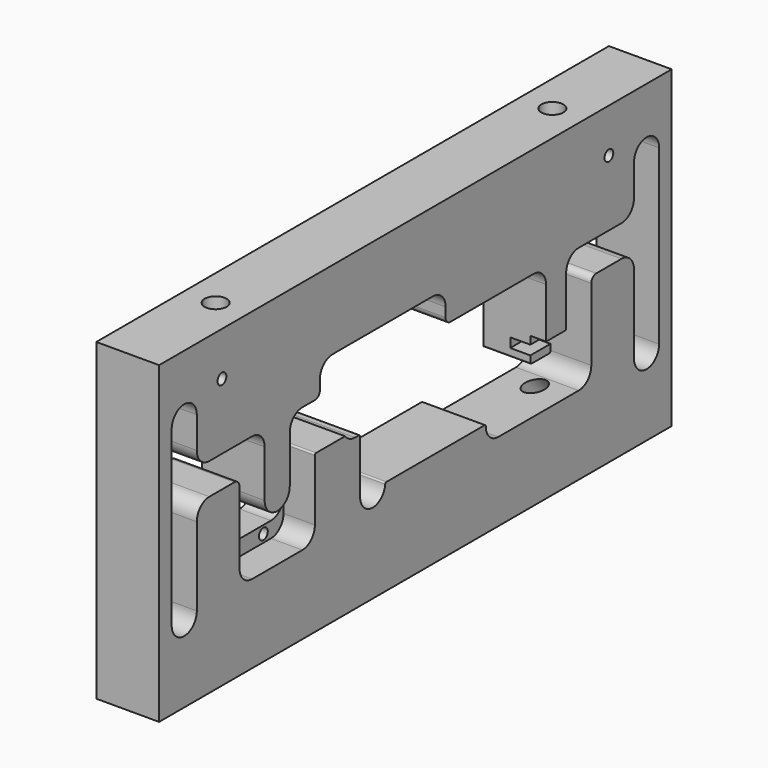
from build123d import *

# Parameters (mm, degrees)
F0_W      = 204
F0_H      = 100
F0_R      = 1.75
F1_DEPTH  = 20
F3_D      = 3.5
F3_DEPTH  = 30
F3_TIP    = 1.0515060833
F5_D      = 7
F5_DEPTH  = 25
F5_TIP    = 2.1030121666
F7_D      = 6
F7_DEPTH  = 27
F7_TIP    = 1.8025818571
F9_R      = 3
F10_DEPTH = 60
F12_D     = 8.5
F12_DEPTH = 15
F12_TIP   = 2.5536576309
F13_DEPTH = 10
F14_W     = 8
F14_H     = 2.5
F14_H_2   = 3
F15_DEPTH = 5
F16_DEPTH = 11.4
F17_R     = 0.5
F18_R     = 0.5
F19_R     = 0.49999


# Not quite as in the source:
# - a fillet or chamfer is up to 0.001 mm smaller than in the source, because OpenCascade refuses the exact size


with BuildPart() as f1:
    # F0 (on Right) → F1 (new body)
    with BuildSketch(Plane.YZ):
        with Locations((-102, 50)):
            Rectangle(F0_W, F0_H)
        with Locations((-179, 86)):
            Circle(F0_R, mode=Mode.SUBTRACT)
        with BuildLine():
            Line((-184, 65), (-167, 65))
            ThreePointArc((-167, 65), (-163.4644660941, 63.5355339059), (-162, 60))
            Line((-162, 60), (-162, 45))
            ThreePointArc((-162, 45), (-157, 40), (-152, 45))
            Line((-152, 45), (-152, 60))
            ThreePointArc((-152, 60), (-150.5355339059, 63.5355339059), (-147, 65))
            Line((-147, 65), (-142, 65))
            ThreePointArc((-142, 65), (-140.5857864376, 65.5857864376), (-140, 67))
            Line((-140, 67), (-140, 70))
            ThreePointArc((-140, 70), (-138.5355339059, 73.5355339059), (-135, 75))
            Line((-135, 75), (-95, 75))
            ThreePointArc((-95, 75), (-91.4644660941, 73.5355339059), (-90, 70))
            Line((-90, 70), (-90, 67))
            ThreePointArc((-90, 67), (-89.4142135624, 65.5857864376), (-88, 65))
            Line((-88, 65), (-55, 65))
            ThreePointArc((-55, 65), (-51.4644660941, 63.5355339059), (-50, 60))
            Line((-50, 60), (-50, 36.5))
            ThreePointArc((-50, 36.5), (-49.8535533906, 36.1464466094), (-49.5, 36))
            Line((-49.5, 36), (-42.5, 36))
            ThreePointArc((-42.5, 36), (-42.1464466094, 36.1464466094), (-42, 36.5))
            Line((-42, 36.5), (-42, 60))
            ThreePointArc((-42, 60), (-40.5355339059, 63.5355339059), (-37, 65))
            Line((-37, 65), (-20, 65))
            ThreePointArc((-20, 65), (-16.4644660941, 66.4644660941), (-15, 70))
            Line((-15, 70), (-15, 80))
            ThreePointArc((-15, 80), (-10, 85), (-5, 80))
            Line((-5, 80), (-5, 25))
            ThreePointArc((-5, 25), (-10, 20), (-15, 25))
            Line((-15, 25), (-15, 50))
            ThreePointArc((-15, 50), (-16.4644660941, 53.5355339059), (-20, 55))
            Line((-20, 55), (-30, 55))
            ThreePointArc((-30, 55), (-31.4142135624, 54.4142135624), (-32, 53))
            Line((-32, 53), (-32, 30))
            ThreePointArc((-32, 30), (-33.4644660941, 26.4644660941), (-37, 25))
            Line((-37, 25), (-69, 25))
            ThreePointArc((-69, 25), (-72.5355339059, 26.4644660941), (-74, 30))
            Line((-74, 30), (-74, 30.5))
            Line((-74, 30.5), (-114, 30.5))
            ThreePointArc((-114, 30.5), (-119, 25.5), (-124, 30.5))
            Line((-124, 30.5), (-124, 48))
            Line((-124, 48), (-126, 48))
            ThreePointArc((-126, 48), (-128.2360679775, 48.527864045), (-130, 50))
            Line((-130, 50), (-141.5, 50))
            ThreePointArc((-141.5, 50), (-141.8535533906, 49.8535533906), (-142, 49.5))
            Line((-142, 49.5), (-142, 35))
            Line((-142, 35), (-142, 30))
            ThreePointArc((-142, 30), (-143.4644660941, 26.4644660941), (-147, 25))
            Line((-147, 25), (-167, 25))
            ThreePointArc((-167, 25), (-170.5355339059, 26.4644660941), (-172, 30))
            Line((-172, 30), (-172, 35))
            Line((-172, 35), (-172, 53))
            ThreePointArc((-172, 53), (-172.5857864376, 54.4142135624), (-174, 55))
            Line((-174, 55), (-184, 55))
            ThreePointArc((-184, 55), (-187.5355339059, 53.5355339059), (-189, 50))
            Line((-189, 50), (-189, 25))
            ThreePointArc((-189, 25), (-194, 20), (-199, 25))
            Line((-199, 25), (-199, 80))
            ThreePointArc((-199, 80), (-194, 85), (-189, 80))
            Line((-189, 80), (-189, 70))
            ThreePointArc((-189, 70), (-187.5355339059, 66.4644660941), (-184, 65))
        make_face(mode=Mode.SUBTRACT)
        with Locations((-25, 86)):
            Circle(F0_R, mode=Mode.SUBTRACT)
    extrude(amount=F1_DEPTH)

    # F3
    with Locations(Plane(origin=(0, 0, 0), x_dir=(1, 0, 0), z_dir=(0, 0, -1))):
        with Locations((10, 119)):
            Hole(F3_D / 2, depth=F3_DEPTH)
            with Locations((0, 0, -(F3_DEPTH + F3_TIP / 2))):  # 118° drill point
                Cone(0, F3_D / 2, F3_TIP, mode=Mode.SUBTRACT)

    # F5
    with Locations(Plane.XY.offset(100)):
        with Locations((10, -169), (10, -35)):
            Hole(F5_D / 2, depth=F5_DEPTH)
            with Locations((0, 0, -(F5_DEPTH + F5_TIP / 2))):  # 118° drill point
                Cone(0, F5_D / 2, F5_TIP, mode=Mode.SUBTRACT)

    # F7
    with Locations(Plane(origin=(0, 0, 0), x_dir=(-1, 0, 0), z_dir=(0, 1, 0))):
        with Locations((-10, 10)):
            Hole(F7_D / 2, depth=F7_DEPTH)
            with Locations((0, 0, -(F7_DEPTH + F7_TIP / 2))):  # 118° drill point
                Cone(0, F7_D / 2, F7_TIP, mode=Mode.SUBTRACT)

    # F9 (on face) → F10 (cut)
    with BuildSketch(Plane(origin=(0, 0, 0), x_dir=(1, 0, 0), z_dir=(0, -0.7071067812, 0.7071067812))):
        with Locations((10, -12)):
            Circle(F9_R)
    extrude(amount=F10_DEPTH, mode=Mode.SUBTRACT)

    # F12
    with Locations(Plane(origin=(0, 0, 0), x_dir=(1, 0, 0), z_dir=(0, 0, -1))):
        with Locations((10, 162), (10, 42)):
            Hole(F12_D / 2, depth=F12_DEPTH)
            with Locations((0, 0, -(F12_DEPTH + F12_TIP / 2))):  # 118° drill point
                Cone(0, F12_D / 2, F12_TIP, mode=Mode.SUBTRACT)

    # F0 (on Right) → F13 (join)
    with BuildSketch(Plane.YZ):
        with BuildLine():
            ThreePointArc((-167, 30), (-170.5355339059, 31.4644660941), (-172, 35))
            Line((-172, 35), (-172, 30))
            ThreePointArc((-172, 30), (-170.5355339059, 26.4644660941), (-167, 25))
            Line((-167, 25), (-147, 25))
            ThreePointArc((-147, 25), (-143.4644660941, 26.4644660941), (-142, 30))
            Line((-142, 30), (-142, 35))
            ThreePointArc((-142, 35), (-143.4644660941, 31.4644660941), (-147, 30))
            Line((-147, 30), (-167, 30))
        make_face()
        with Locations((-164, 27.5)):
            Circle(F0_R, mode=Mode.SUBTRACT)
        with Locations((-150, 27.5)):
            Circle(F0_R, mode=Mode.SUBTRACT)
    extrude(amount=F13_DEPTH)

    # F14 (on face) → F15 (cut)
    with BuildSketch(Plane.YZ.offset(20)):
        with Locations((-46, 37.25)):
            Rectangle(F14_W, F14_H)
        with Locations((-46, 40)):
            Rectangle(F14_W, F14_H_2)
        with Locations((-46, 42.75)):
            Rectangle(F14_W, F14_H)
    extrude(amount=-F15_DEPTH, mode=Mode.SUBTRACT)

    # F14 (on face) → F16 (cut)
    with BuildSketch(Plane.YZ.offset(20)):
        with Locations((-46, 40)):
            Rectangle(F14_W, F14_H_2)
    extrude(amount=-F16_DEPTH, mode=Mode.SUBTRACT)

    # F17
    f17_edges = [f1.edges().sort_by_distance(p)[0] for p in [
        (10, -124, 48),
    ]]
    fillet(f17_edges, radius=F17_R)

    # F18
    f18_edges = [f1.edges().sort_by_distance(p)[0] for p in [
        (10, -114, 30.5),
    ]]
    fillet(f18_edges, radius=F18_R)

    # F19 (radius 0.5 in the source; OpenCascade refuses exactly that, so slightly less here)
    f19_edges = [f1.edges().sort_by_distance(p)[0] for p in [
        (10, -74, 30.5),
    ]]
    fillet(f19_edges, radius=F19_R)


solid = f1.part
